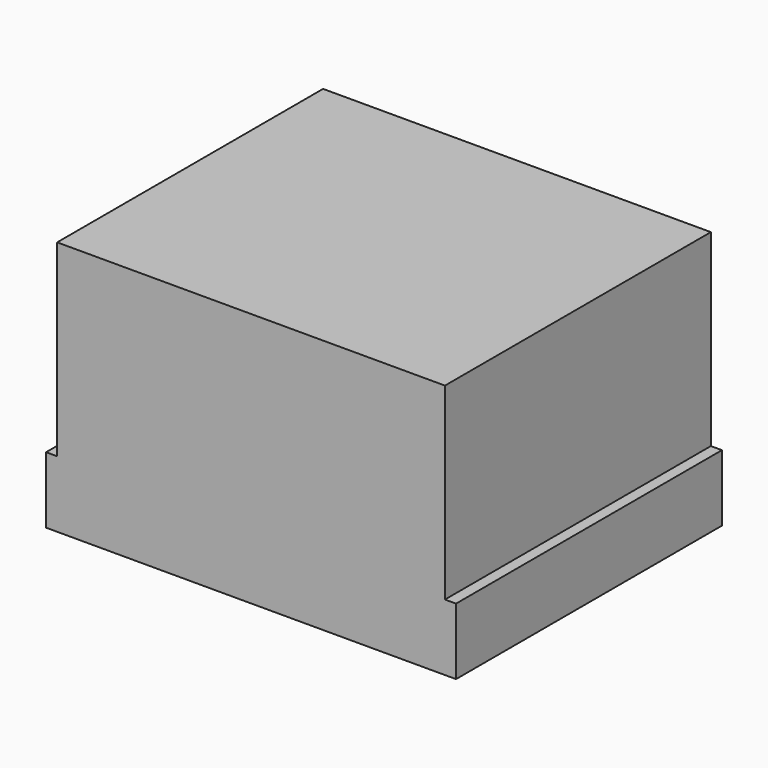
from build123d import *

# Parameters (mm, degrees)
F0_W     = 7
F0_H     = 17
F0_W_2   = 37
F0_H_2   = 2
F1_DEPTH = 30


# Not quite as in the source:
# - a feature names something its author has since deleted; it is built from what else it names


with BuildPart() as f1:
    # F0 (on Front) → F1 (new body)
    with BuildSketch(Plane.XZ):
        with Locations((31.5, 8.5)):
            Rectangle(F0_W, F0_H)
        with Locations((3.5, 8.5)):
            Rectangle(F0_W, F0_H)
        with Locations((17.5, 8.5)):
            Rectangle(F0_W, F0_H)
        with Locations((17.5, -3)):
            Rectangle(F0_W_2, F0_H_2)
        with Locations((10.5, 8.5)):
            Rectangle(F0_W, F0_H)
        Polygon((36, -4), (-1, -4), (-1, -6), (0, -6), (35, -6), (36, -6), align=None)
        Polygon((7, 0), (0, 0), (-1, 0), (-1, -2), (36, -2), (36, 0), (35, 0), (28, 0), (21, 0), (14, 0), align=None)
        with Locations((24.5, 8.5)):
            Rectangle(F0_W, F0_H)
    extrude(amount=F1_DEPTH)


solid = f1.part
